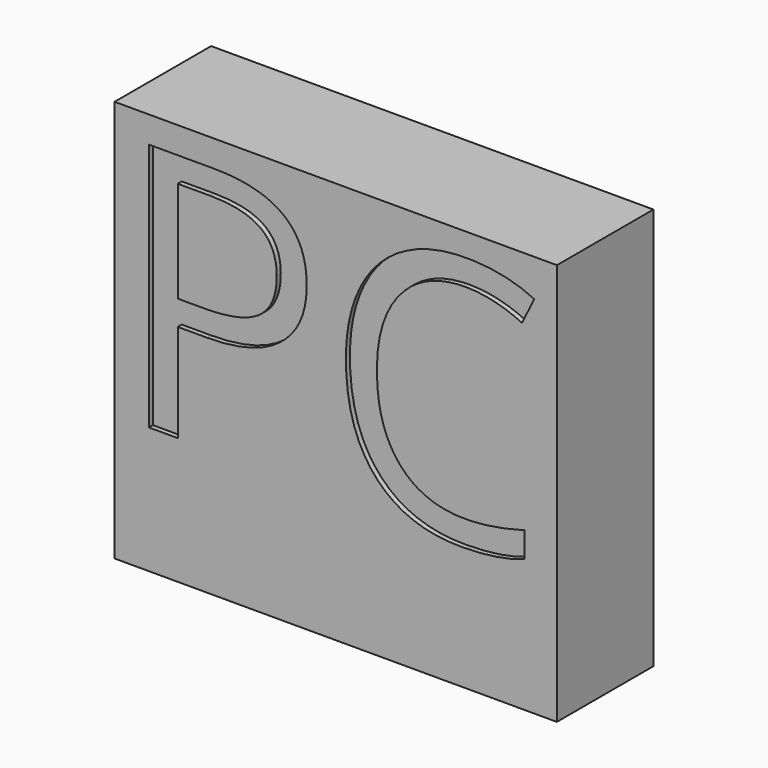
from build123d import *

# Parameters (mm, degrees)
F0_W         = 120
F0_H         = 400
F1_DEPTH     = 440
F2_TEXT_SIZE = 347.011706716
F3_DEPTH     = 5


# Not quite as in the source:
# - Text() gives the source's letters only with a copy of the font that has no kerning and outlines rounded to 1/6400 em; it was checked with that copy


with BuildPart() as f1:
    # F0 (on Right) → F1 (new body)
    with BuildSketch(Plane.YZ):
        with Locations((99.1080081463, 240.8544242382)):
            Rectangle(F0_W, F0_H)
    extrude(amount=F1_DEPTH)

    # F2 (on face) → F3 (cut)
    with BuildSketch(Plane.XZ.offset(-39.1080081463)):
        with Locations((0, 166.7309987975)):
            Text('PC', F2_TEXT_SIZE, font='Open Sans', text_align=(TextAlign.LEFT, TextAlign.BOTTOM))
    extrude(amount=-F3_DEPTH, mode=Mode.SUBTRACT)


solid = f1.part
